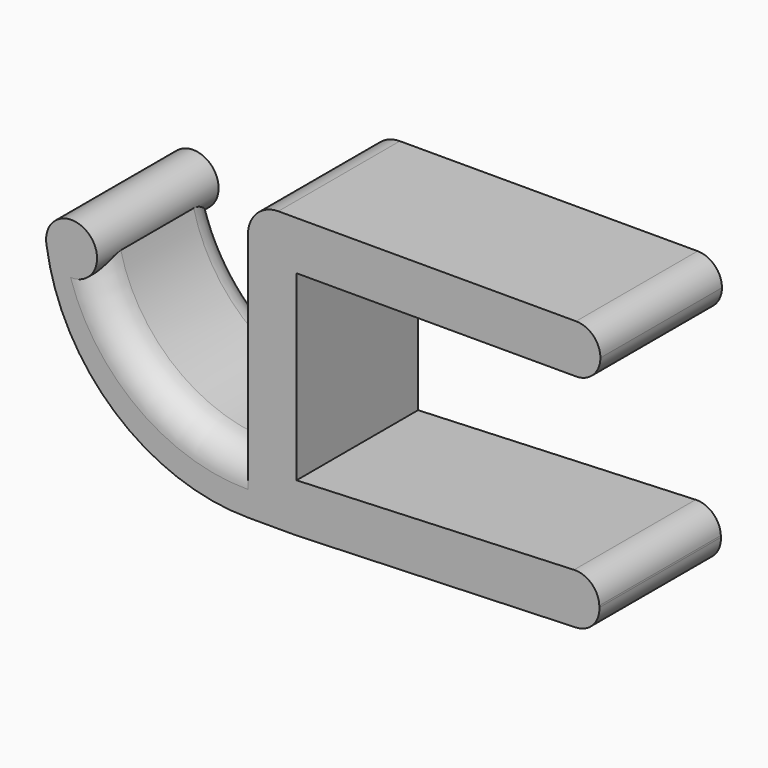
from build123d import *

# Parameters (mm, degrees)
F0_W     = 50
F0_H     = 8
F1_DEPTH = 25
F2_R     = 3.99999
F3_R     = 5


# Not quite as in the source:
# - a fillet or chamfer is up to 0.001 mm smaller than in the source, because OpenCascade refuses the exact size


with BuildPart() as f1:
    # F0 (on Front) → F1 (new body)
    with BuildSketch(Plane.XZ):
        with BuildLine():
            ThreePointArc((-33.1246824974, 28.5893382254), (-21.8780417926, 8.1356985419), (0, 0))
            Line((0, 0), (0, 9.0772153518))
            ThreePointArc((0, 9.0772153518), (-15.8507153639, 14.5046379043), (-24.9239347471, 28.5893382254))
            ThreePointArc((-24.9239347471, 28.5893382254), (-29.0243086222, 33.6818376736), (-33.1246824974, 28.5893382254))
        make_face()
        with Locations((33, 42)):
            Rectangle(F0_W, F0_H)
        Polygon((57.6595105231, 10.0428396836), (8, 8), (57.743546671, 8), align=None)
        Polygon((0, 9.0772153518), (0, 0), (8, 0), (8, 8), (8, 38), (8, 46), (0, 46), align=None)
        Polygon((8, 8), (8, 0), (58, 1.7658608791), (57.743546671, 8), align=None)
    extrude(amount=F1_DEPTH)

    # F2 (radius 4 in the source; OpenCascade refuses exactly that, so slightly less here)
    f2_edges = [f1.edges().sort_by_distance(p)[0] for p in [
        (58, -12.5, 46),
        (58, -12.5, 38),
        (57.659511, -12.5, 10.04284),
        (58, -12.5, 1.765861),
    ]]
    fillet(f2_edges, radius=F2_R)

    # F3
    f3_edges = [f1.edges().sort_by_distance(p)[0] for p in [
        (-15.850715, -25, 14.504638),
        (-15.850715, 0, 14.504638),
        (0, -12.5, 46),
    ]]
    fillet(f3_edges, radius=F3_R)


solid = f1.part
